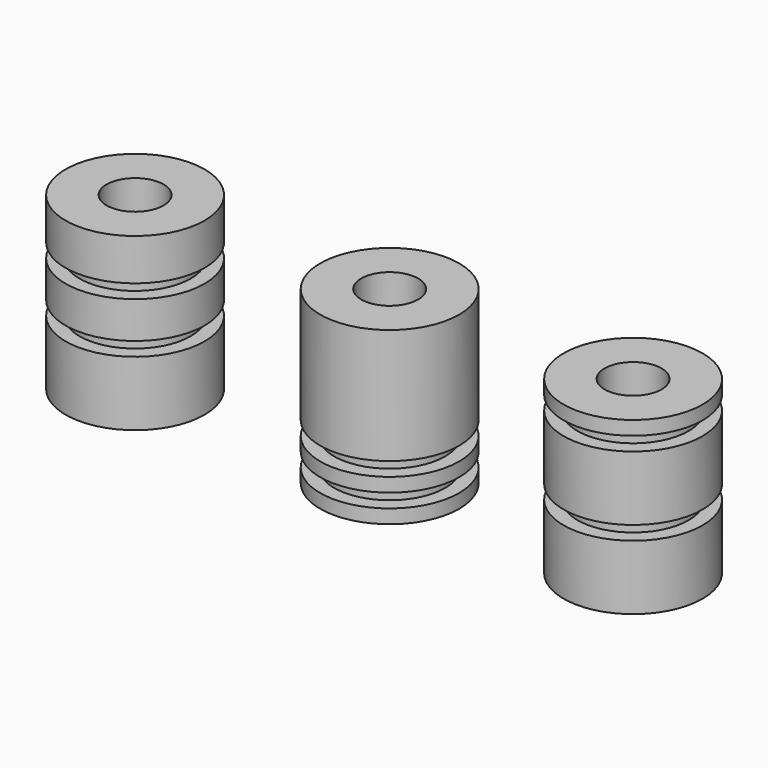
from build123d import *

# Parameters (mm, degrees)
F0_R      = 5
F0_R_2    = 2.05
F1_DEPTH  = 1
F2_R      = 4
F2_R_2    = 2.05
F3_DEPTH  = 1
F4_R      = 5
F4_R_2    = 4
F4_R_3    = 2.05
F5_DEPTH  = 1
F6_R      = 4
F6_R_2    = 2.05
F7_DEPTH  = 1
F8_R      = 5
F8_R_2    = 4
F8_R_3    = 2.05
F9_DEPTH  = 8.3
F10_DEPTH = 4.65
F11_R     = 4
F11_R_2   = 2.05
F12_DEPTH = 1
F13_R     = 5
F13_R_2   = 4
F13_R_3   = 2.05
F14_DEPTH = 4.65
F15_DEPTH = 4.65
F16_R     = 4
F16_R_2   = 2.05
F17_DEPTH = 1
F18_R     = 5
F18_R_2   = 4
F18_R_3   = 2.05
F19_DEPTH = 2.65
F20_R     = 4
F20_R_2   = 2.05
F21_DEPTH = 1
F22_R     = 5
F22_R_2   = 4
F22_R_3   = 2.05
F23_DEPTH = 3
F24_R     = 4
F24_R_2   = 2.05
F25_DEPTH = 1
F26_R     = 5
F26_R_2   = 4
F26_R_3   = 2.05
F27_DEPTH = 1


with BuildPart() as f1:
    # F0 (on Top) → F1 (new body)
    with BuildSketch(Plane.XY):
        with Locations((0.204080643, -0.5602314472)):
            Circle(F0_R)
        with Locations((0.204080643, -0.5602314472)):
            Circle(F0_R_2, mode=Mode.SUBTRACT)
    extrude(amount=F1_DEPTH)

    # F2 (on face) → F3 (join)
    with BuildSketch(Plane.XY.offset(1)):
        with Locations((0.204080643, -0.5602314472)):
            Circle(F2_R)
        with Locations((0.204080643, -0.5602314472)):
            Circle(F2_R_2, mode=Mode.SUBTRACT)
    extrude(amount=F3_DEPTH)

    # F4 (on face) → F5 (join)
    with BuildSketch(Plane.XY.offset(2)):
        with Locations((0.204080643, -0.5602314472)):
            Circle(F4_R)
        with Locations((0.204080643, -0.5602314472)):
            Circle(F4_R_2, mode=Mode.SUBTRACT)
        with Locations((0.204080643, -0.5602314472)):
            Circle(F4_R_2)
        with Locations((0.204080643, -0.5602314472)):
            Circle(F4_R_3, mode=Mode.SUBTRACT)
    extrude(amount=F5_DEPTH)

    # F6 (on face) → F7 (join)
    with BuildSketch(Plane.XY.offset(3)):
        with Locations((0.204080643, -0.5602314472)):
            Circle(F6_R)
        with Locations((0.204080643, -0.5602314472)):
            Circle(F6_R_2, mode=Mode.SUBTRACT)
    extrude(amount=F7_DEPTH)

    # F8 (on face) → F9 (join)
    with BuildSketch(Plane.XY.offset(4)):
        with Locations((0.204080643, -0.5602314472)):
            Circle(F8_R)
        with Locations((0.204080643, -0.5602314472)):
            Circle(F8_R_2, mode=Mode.SUBTRACT)
        with Locations((0.204080643, -0.5602314472)):
            Circle(F8_R_2)
        with Locations((0.204080643, -0.5602314472)):
            Circle(F8_R_3, mode=Mode.SUBTRACT)
    extrude(amount=F9_DEPTH)


with BuildPart() as f10:
    # F0 (on Top) → F10 (new body)
    with BuildSketch(Plane.XY):
        with Locations((17.7169614471, -0.5602314472)):
            Circle(F0_R)
        with Locations((17.7169614471, -0.5602314472)):
            Circle(F0_R_2, mode=Mode.SUBTRACT)
    extrude(amount=F10_DEPTH)

    # F11 (on face) → F12 (join)
    with BuildSketch(Plane.XY.offset(4.65)):
        with Locations((17.7169614471, -0.5602314472)):
            Circle(F11_R)
        with Locations((17.7169614471, -0.5602314472)):
            Circle(F11_R_2, mode=Mode.SUBTRACT)
    extrude(amount=F12_DEPTH)

    # F13 (on face) → F14 (join)
    with BuildSketch(Plane.XY.offset(5.65)):
        with Locations((17.7169614471, -0.5602314472)):
            Circle(F13_R)
        with Locations((17.7169614471, -0.5602314472)):
            Circle(F13_R_2, mode=Mode.SUBTRACT)
        with Locations((17.7169614471, -0.5602314472)):
            Circle(F13_R_2)
        with Locations((17.7169614471, -0.5602314472)):
            Circle(F13_R_3, mode=Mode.SUBTRACT)
    extrude(amount=F14_DEPTH)

    # F24 (on face) → F25 (join)
    with BuildSketch(Plane.XY.offset(10.3)):
        with Locations((17.7169614471, -0.5602314472)):
            Circle(F24_R)
        with Locations((17.7169614471, -0.5602314472)):
            Circle(F24_R_2, mode=Mode.SUBTRACT)
    extrude(amount=F25_DEPTH)

    # F26 (on face) → F27 (join)
    with BuildSketch(Plane.XY.offset(11.3)):
        with Locations((17.7169614471, -0.5602314472)):
            Circle(F26_R)
        with Locations((17.7169614471, -0.5602314472)):
            Circle(F26_R_2, mode=Mode.SUBTRACT)
        with Locations((17.7169614471, -0.5602314472)):
            Circle(F26_R_2)
        with Locations((17.7169614471, -0.5602314472)):
            Circle(F26_R_3, mode=Mode.SUBTRACT)
    extrude(amount=F27_DEPTH)


with BuildPart() as f15:
    # F0 (on Top) → F15 (new body)
    with BuildSketch(Plane.XY):
        with Locations((-18.1162464432, -0.5602314472)):
            Circle(F0_R)
        with Locations((-18.1162464432, -0.5602314472)):
            Circle(F0_R_2, mode=Mode.SUBTRACT)
    extrude(amount=F15_DEPTH)

    # F16 (on face) → F17 (join)
    with BuildSketch(Plane.XY.offset(4.65)):
        with Locations((-18.1162464432, -0.5602314472)):
            Circle(F16_R)
        with Locations((-18.1162464432, -0.5602314472)):
            Circle(F16_R_2, mode=Mode.SUBTRACT)
    extrude(amount=F17_DEPTH)

    # F18 (on face) → F19 (join)
    with BuildSketch(Plane.XY.offset(5.65)):
        with Locations((-18.1162464432, -0.5602314472)):
            Circle(F18_R)
        with Locations((-18.1162464432, -0.5602314472)):
            Circle(F18_R_2, mode=Mode.SUBTRACT)
        with Locations((-18.1162464432, -0.5602314472)):
            Circle(F18_R_2)
        with Locations((-18.1162464432, -0.5602314472)):
            Circle(F18_R_3, mode=Mode.SUBTRACT)
    extrude(amount=F19_DEPTH)

    # F20 (on face) → F21 (join)
    with BuildSketch(Plane.XY.offset(8.3)):
        with Locations((-18.1162464432, -0.5602314472)):
            Circle(F20_R)
        with Locations((-18.1162464432, -0.5602314472)):
            Circle(F20_R_2, mode=Mode.SUBTRACT)
    extrude(amount=F21_DEPTH)

    # F22 (on face) → F23 (join)
    with BuildSketch(Plane.XY.offset(9.3)):
        with Locations((-18.1162464432, -0.5602314472)):
            Circle(F22_R)
        with Locations((-18.1162464432, -0.5602314472)):
            Circle(F22_R_2, mode=Mode.SUBTRACT)
        with Locations((-18.1162464432, -0.5602314472)):
            Circle(F22_R_2)
        with Locations((-18.1162464432, -0.5602314472)):
            Circle(F22_R_3, mode=Mode.SUBTRACT)
    extrude(amount=F23_DEPTH)


solid = Compound([f1.part, f10.part, f15.part])
